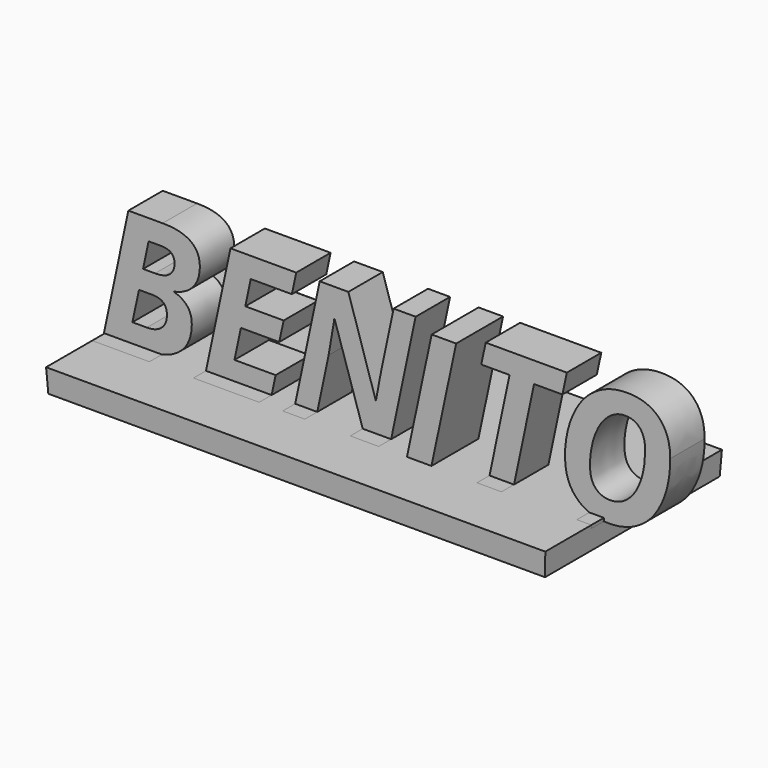
from build123d import *

# Parameters (mm, degrees)
F0_W         = 127.0725689828
F0_H         = 55.8486226946
F1_DEPTH     = 6
F1_TAPER     = -3
F2_TEXT_SIZE = 42.1051246425
F3_DEPTH     = 15
F4_DEPTH     = 4


# Not quite as in the source:
# - Text() gives the source's letters only with a copy of the font that has no kerning and outlines rounded to 1/6400 em; it was checked with that copy


with BuildPart() as f1:
    # F0 (on Top) → F1 (new body)
    with BuildSketch(Plane.XY):
        with Locations((2.6256311685, -1.4981189743)):
            Rectangle(F0_W, F0_H)
    extrude(amount=F1_DEPTH, taper=F1_TAPER)

    # F2 (on Front) → F3 (join)
    with BuildSketch(Plane.XZ):
        with Locations((-62.6068824228, 5.5614031106)):
            Text('BENITO', F2_TEXT_SIZE, font='Open Sans', font_style=FontStyle.BOLDITALIC, text_align=(TextAlign.LEFT, TextAlign.BOTTOM))
    extrude(amount=F3_DEPTH)

    # F4 (cut): faces of the model
    f4_faces = [f1.faces().sort_by_distance(p)[0] for p in [
        (-48.9311599907, -15, 20.5698286651),
        (-25.2100325698, -15, 20.9929452609),
        (2.9289353838, -15, 20.8222461824),
        (44.2331906394, -15, 24.3691818739),
        (62.2318007871, -15, 31.4619998371),
    ]]
    extrude(f4_faces, amount=-F4_DEPTH, mode=Mode.SUBTRACT)


solid = f1.part
